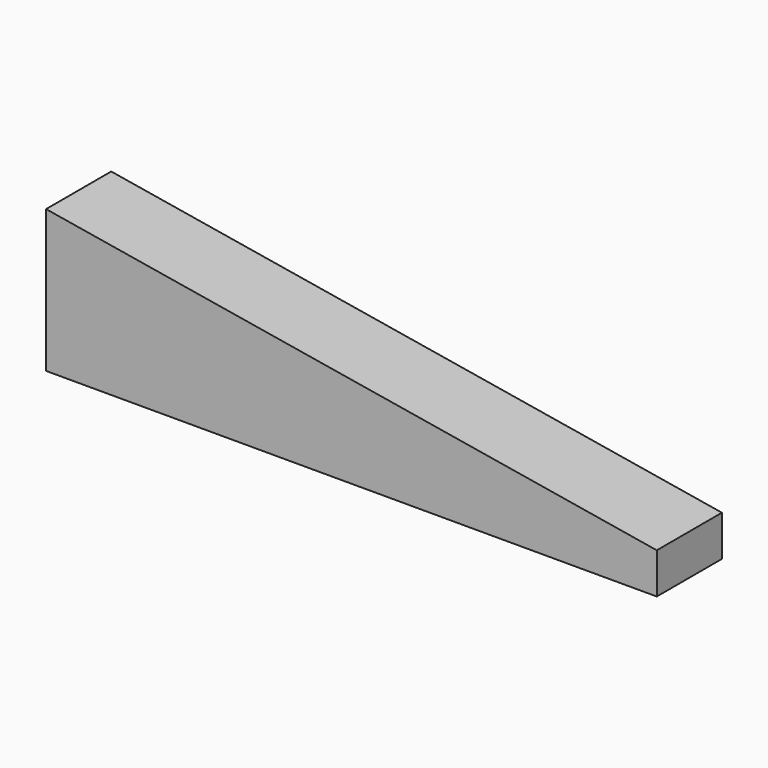
from build123d import *

# Parameters (mm, degrees)
F1_DEPTH = 40


# Not quite as in the source:
# - the program builds the solid bodies; features that only make, move or delete a surface that nothing else refers to are left out


with BuildPart() as f1:
    # F0 (on Front) → F1 (new body)
    with BuildSketch(Plane.XZ):
        Polygon((0, 70), (0, 0), (300, 0), (300, 20), align=None)
    extrude(amount=F1_DEPTH)


solid = f1.part
